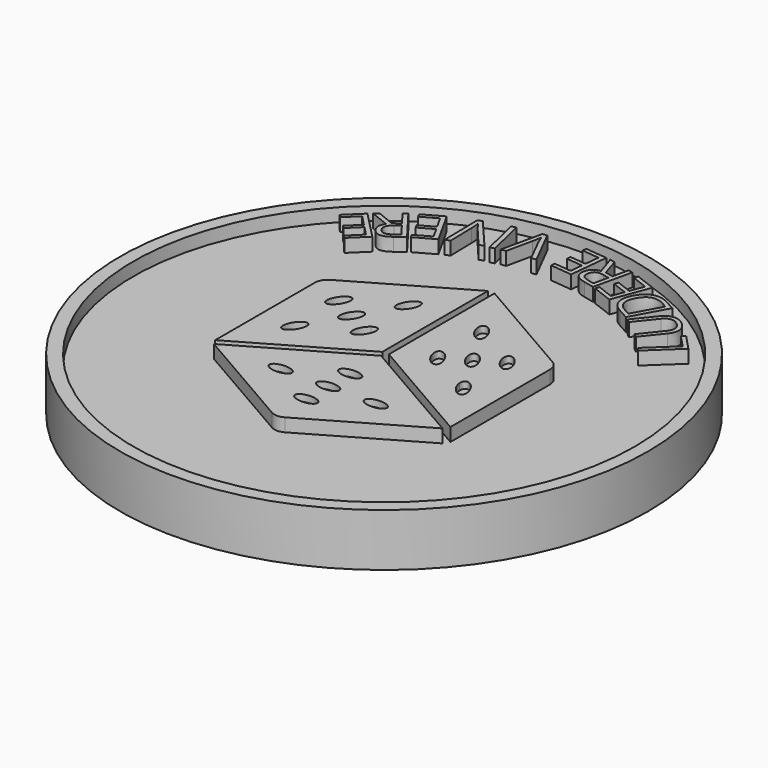
from build123d import *

# Parameters (mm, degrees)
F0_R          = 10
F1_DEPTH      = 2
F2_R          = 9.5
F3_DEPTH      = 0.5
F4_R          = 9.25
F5_DEPTH      = 0.5
F7_DEPTH      = 0.5
F9_DEPTH      = 0.25
F10_TEXT_SIZE = 2.0833333333
F11_DEPTH     = 0.5
F13_TEXT_SIZE = 15.2777777778
F14_DEPTH     = 0.5


# Not quite as in the source:
# - Text() gives the source's letters only with a copy of the font that has no kerning and outlines rounded to 1/6400 em; it was checked with that copy


with BuildPart() as f1:
    # F0 (on Top) → F1 (new body)
    with BuildSketch(Plane.XY):
        Circle(F0_R)
    extrude(amount=F1_DEPTH)

    # F2 (on face) → F3 (cut)
    with BuildSketch(Plane.XY.offset(2)):
        Circle(F2_R)
    extrude(amount=-F3_DEPTH, mode=Mode.SUBTRACT)

    # F4 (on face) → F5 (cut)
    with BuildSketch(Plane(origin=(0, 0, 0), x_dir=(1, 0, 0), z_dir=(0, 0, -1))):
        Circle(F4_R)
    extrude(amount=-F5_DEPTH, mode=Mode.SUBTRACT)

    # F6 (on face) → F7 (join, through all)
    with BuildSketch(Plane.XY.offset(2)):
        with BuildLine():
            Line((-0.125, 0.0721687836), (-0.125, 5.0721687836))
            Line((-0.125, 5.0721687836), (-4.2051270189, 2.7165063509))
            ThreePointArc((-4.2051270189, 2.7165063509), (-4.3881397208, 2.5334936491), (-4.4551270189, 2.2834936491))
            Line((-4.4551270189, 2.2834936491), (-4.4551270189, -2.4278312164))
            Line((-4.4551270189, -2.4278312164), (-0.125, 0.0721687836))
        make_face()
        with BuildLine():
            Line((0, -0.1443375673), (-4.3301270189, -2.6443375673))
            Line((-4.3301270189, -2.6443375673), (-0.25, -5))
            ThreePointArc((-0.25, -5), (0, -5.0669872981), (0.25, -5))
            Line((0.25, -5), (4.3301270189, -2.6443375673))
            Line((4.3301270189, -2.6443375673), (0, -0.1443375673))
        make_face()
        with BuildLine():
            Line((0.125, 0.0721687836), (4.4551270189, -2.4278312164))
            Line((4.4551270189, -2.4278312164), (4.4551270189, 2.2834936491))
            ThreePointArc((4.4551270189, 2.2834936491), (4.3881397208, 2.5334936491), (4.2051270189, 2.7165063509))
            Line((4.2051270189, 2.7165063509), (0.125, 5.0721687836))
            Line((0.125, 5.0721687836), (0.125, 0.0721687836))
        make_face()
    extrude(amount=-F7_DEPTH)

    # F8 (on face) → F9 (cut)
    with BuildSketch(Plane.XY.offset(2)):
        with BuildLine():
            add(Edge.make_bspline(
                [(-0.4265724856, -2.6443375673), (-0.4265724856, -3.0189013437), (0.2132862428, -2.8316194555), (0.8531449712, -2.6443375673), (0.2132862428, -2.4570556791), (-0.4265724856, -2.2697737909), (-0.4265724856, -2.6443375673)],
                knots=[0, 0, 0, 2.0943951024, 2.0943951024, 4.1887902048, 4.1887902048, 6.2831853072, 6.2831853072, 6.2831853072], degree=2, weights=[1, 0.5, 1, 0.5, 1, 0.5, 1]))
        make_face()
        with BuildLine():
            add(Edge.make_bspline(
                [(1.3734275144, -2.6443375673), (1.3734275144, -3.0189013437), (2.0132862428, -2.8316194555), (2.6531449712, -2.6443375673), (2.0132862428, -2.4570556791), (1.3734275144, -2.2697737909), (1.3734275144, -2.6443375673)],
                knots=[0, 0, 0, 2.0943951024, 2.0943951024, 4.1887902048, 4.1887902048, 6.2831853072, 6.2831853072, 6.2831853072], degree=2, weights=[1, 0.5, 1, 0.5, 1, 0.5, 1]))
        make_face()
        with BuildLine():
            add(Edge.make_bspline(
                [(-1.5185417438, -2.4818375673), (-2.2265724856, -2.1666585057), (-2.2265724856, -2.6443375673)],
                knots=[3.9918185291, 3.9918185291, 3.9918185291, 6.2831853072, 6.2831853072, 6.2831853072], degree=2, weights=[1, 0.4124236698, 1]))
            add(Edge.make_bspline(
                [(-2.2265724856, -2.6443375673), (-2.2265724856, -2.9796236254), (-1.6240714101, -2.8413437189), (-1.0215703345, -2.7030638124), (-1.5185417438, -2.4818375673)],
                knots=[0, 0, 0, 1.9959092646, 1.9959092646, 3.9918185291, 3.9918185291, 3.9918185291], degree=2, weights=[1, 0.5420222921, 1, 0.5420222921, 1]))
        make_face()
        with BuildLine():
            add(Edge.make_bspline(
                [(-0.4265724856, -1.6051070828), (-0.4265724856, -1.7030096523), (-0.2814582562, -1.7676070828)],
                knots=[0, 0, 0, 0.8502258755, 0.8502258755, 0.8502258755], degree=2, weights=[1, 0.9109921606, 1]))
            add(Edge.make_bspline(
                [(-0.2814582562, -1.7676070828), (0.1270605196, -1.9494587409), (0.378292689, -1.705041847), (0.6295248585, -1.460624953), (0.1014761864, -1.3950606558), (-0.4265724856, -1.3294963586), (-0.4265724856, -1.6051070828)],
                knots=[0.8502258755, 0.8502258755, 0.8502258755, 2.6612123527, 2.6612123527, 4.47219883, 4.47219883, 6.2831853072, 6.2831853072, 6.2831853072], degree=2, weights=[1, 0.6172976096, 1, 0.6172976096, 1, 0.6172976096, 1]))
        make_face()
        with BuildLine():
            add(Edge.make_bspline(
                [(-0.4265724856, -3.6835680518), (-0.4265724856, -4.0581318282), (0.2132862428, -3.87084994), (0.8531449712, -3.6835680518), (0.2132862428, -3.4962861636), (-0.4265724856, -3.3090042754), (-0.4265724856, -3.6835680518)],
                knots=[0, 0, 0, 2.0943951024, 2.0943951024, 4.1887902048, 4.1887902048, 6.2831853072, 6.2831853072, 6.2831853072], degree=2, weights=[1, 0.5, 1, 0.5, 1, 0.5, 1]))
        make_face()
        with BuildLine():
            add(Edge.make_bspline(
                [(1.6033497523, 0.4331309323), (1.6881358645, 0.482082217), (1.6715217657, 0.6400535414)],
                knots=[0, 0, 0, 0.8502258755, 0.8502258755, 0.8502258755], degree=2, weights=[1, 0.9109921606, 1]))
            add(Edge.make_bspline(
                [(1.6715217657, 0.6400535414), (1.6247505334, 1.0847670082), (1.2874632095, 1.1801320022), (0.9501758855, 1.2754969962), (1.1574198745, 0.7854112832), (1.3646638636, 0.2953255702), (1.6033497523, 0.4331309323)],
                knots=[0.8502258755, 0.8502258755, 0.8502258755, 2.6612123527, 2.6612123527, 4.47219883, 4.47219883, 6.2831853072, 6.2831853072, 6.2831853072], degree=2, weights=[1, 0.6172976096, 1, 0.6172976096, 1, 0.6172976096, 1]))
        make_face()
        with BuildLine():
            add(Edge.make_bspline(
                [(3.4033497523, -0.6060995522), (3.6937159961, -0.4384565232), (3.2727115465, 0.0141847608), (2.8517070968, 0.4668260447), (2.9086052532, -0.0741769432)],
                knots=[0, 0, 0, 1.9959092646, 1.9959092646, 3.9918185291, 3.9918185291, 3.9918185291], degree=2, weights=[1, 0.5420222921, 1, 0.5420222921, 1]))
            add(Edge.make_bspline(
                [(2.9086052532, -0.0741769432), (2.98966755, -0.844939083), (3.4033497523, -0.6060995522)],
                knots=[3.9918185291, 3.9918185291, 3.9918185291, 6.2831853072, 6.2831853072, 6.2831853072], degree=2, weights=[1, 0.4124236698, 1]))
        make_face()
        with BuildLine():
            add(Edge.make_bspline(
                [(1.6033497523, 2.5115919014), (1.9277314979, 2.6988737896), (1.4456112609, 3.1593667591), (0.9634910239, 3.6198597286), (1.1212295152, 2.9720848709), (1.2789680066, 2.3243100132), (1.6033497523, 2.5115919014)],
                knots=[0, 0, 0, 2.0943951024, 2.0943951024, 4.1887902048, 4.1887902048, 6.2831853072, 6.2831853072, 6.2831853072], degree=2, weights=[1, 0.5, 1, 0.5, 1, 0.5, 1]))
        make_face()
        with BuildLine():
            add(Edge.make_bspline(
                [(3.4033497523, 1.4723614168), (3.7277314979, 1.659643305), (3.2456112609, 2.1201362746), (2.7634910239, 2.5806292441), (2.9212295152, 1.9328543864), (3.0789680066, 1.2850795286), (3.4033497523, 1.4723614168)],
                knots=[0, 0, 0, 2.0943951024, 2.0943951024, 4.1887902048, 4.1887902048, 6.2831853072, 6.2831853072, 6.2831853072], degree=2, weights=[1, 0.5, 1, 0.5, 1, 0.5, 1]))
        make_face()
        with BuildLine():
            add(Edge.make_bspline(
                [(2.5033497523, 0.9527461746), (2.8277314979, 1.1400280628), (2.3456112609, 1.6005210323), (1.8634910239, 2.0610140018), (2.0212295152, 1.4132391441), (2.1789680066, 0.7654642864), (2.5033497523, 0.9527461746)],
                knots=[0, 0, 0, 2.0943951024, 2.0943951024, 4.1887902048, 4.1887902048, 6.2831853072, 6.2831853072, 6.2831853072], degree=2, weights=[1, 0.5, 1, 0.5, 1, 0.5, 1]))
        make_face()
        with BuildLine():
            add(Edge.make_bspline(
                [(-1.1767772667, 1.1719761505), (-1.2615633789, 1.2209274352), (-1.3900635095, 1.1275535414)],
                knots=[0, 0, 0, 0.8502258755, 0.8502258755, 0.8502258755], degree=2, weights=[1, 0.9109921606, 1]))
            add(Edge.make_bspline(
                [(-1.3900635095, 1.1275535414), (-1.751811053, 0.8646917327), (-1.6657558985, 0.5249098447), (-1.5797007439, 0.1851279568), (-1.258896061, 0.6096493726), (-0.938091378, 1.0341707884), (-1.1767772667, 1.1719761505)],
                knots=[0.8502258755, 0.8502258755, 0.8502258755, 2.6612123527, 2.6612123527, 4.47219883, 4.47219883, 6.2831853072, 6.2831853072, 6.2831853072], degree=2, weights=[1, 0.6172976096, 1, 0.6172976096, 1, 0.6172976096, 1]))
        make_face()
        with BuildLine():
            add(Edge.make_bspline(
                [(-1.1767772667, 3.2504371195), (-1.4671435105, 3.4180801486), (-1.6486401364, 2.8271589581), (-1.8301367623, 2.2362377676), (-1.3900635095, 2.5560145105)],
                knots=[0, 0, 0, 1.9959092646, 1.9959092646, 3.9918185291, 3.9918185291, 3.9918185291], degree=2, weights=[1, 0.5420222921, 1, 0.5420222921, 1]))
            add(Edge.make_bspline(
                [(-1.3900635095, 2.5560145105), (-0.7630950645, 3.0115975887), (-1.1767772667, 3.2504371195)],
                knots=[3.9918185291, 3.9918185291, 3.9918185291, 6.2831853072, 6.2831853072, 6.2831853072], degree=2, weights=[1, 0.4124236698, 1]))
        make_face()
        with BuildLine():
            add(Edge.make_bspline(
                [(-2.9767772667, 0.1327456659), (-3.3011590124, 0.3200275541), (-3.4588975037, -0.3277473036), (-3.6166359951, -0.9755221613), (-3.134515758, -0.5150291918), (-2.652395521, -0.0545362223), (-2.9767772667, 0.1327456659)],
                knots=[0, 0, 0, 2.0943951024, 2.0943951024, 4.1887902048, 4.1887902048, 6.2831853072, 6.2831853072, 6.2831853072], degree=2, weights=[1, 0.5, 1, 0.5, 1, 0.5, 1]))
        make_face()
        with BuildLine():
            add(Edge.make_bspline(
                [(-2.9767772667, 2.211206635), (-3.3011590124, 2.3984885232), (-3.4588975037, 1.7507136655), (-3.6166359951, 1.1029388078), (-3.134515758, 1.5634317773), (-2.652395521, 2.0239247468), (-2.9767772667, 2.211206635)],
                knots=[0, 0, 0, 2.0943951024, 2.0943951024, 4.1887902048, 4.1887902048, 6.2831853072, 6.2831853072, 6.2831853072], degree=2, weights=[1, 0.5, 1, 0.5, 1, 0.5, 1]))
        make_face()
        with BuildLine():
            add(Edge.make_bspline(
                [(-2.0767772667, 1.6915913927), (-2.4011590124, 1.8788732809), (-2.5588975037, 1.2310984232), (-2.7166359951, 0.5833235655), (-2.234515758, 1.043816535), (-1.752395521, 1.5043095045), (-2.0767772667, 1.6915913927)],
                knots=[0, 0, 0, 2.0943951024, 2.0943951024, 4.1887902048, 4.1887902048, 6.2831853072, 6.2831853072, 6.2831853072], degree=2, weights=[1, 0.5, 1, 0.5, 1, 0.5, 1]))
        make_face()
    extrude(amount=-F9_DEPTH, mode=Mode.SUBTRACT)

    # F10 (on face) → F11 (join, through all)
    with BuildSketch(Plane.XY.offset(2)):
        with Locations(Location((1.4901733322, 8.8949874364), (0, 0, 174.204199698))):
            Text('E', F10_TEXT_SIZE, font='Open Sans', text_align=(TextAlign.LEFT, TextAlign.BOTTOM))
        with Locations(Location((6.9602849105, 5.7354905649), (0, 0, 133.204199698))):
            Text('L', F10_TEXT_SIZE, font='Open Sans', text_align=(TextAlign.LEFT, TextAlign.BOTTOM))
        with Locations(Location((6.2088700096, 6.5562723689), (0, 0, 141.204199698))):
            Text('U', F10_TEXT_SIZE, font='Open Sans', text_align=(TextAlign.LEFT, TextAlign.BOTTOM))
        with Locations(Location((5.0041574298, 7.5193820274), (0, 0, 151.204199698))):
            Text('D', F10_TEXT_SIZE, font='Open Sans', text_align=(TextAlign.LEFT, TextAlign.BOTTOM))
        with Locations(Location((3.7415890618, 8.2062128505), (0, 0, 159.204199698))):
            Text('E', F10_TEXT_SIZE, font='Open Sans', text_align=(TextAlign.LEFT, TextAlign.BOTTOM))
        with Locations(Location((2.6697508212, 8.6228550543), (0, 0, 167.204199698))):
            Text('R', F10_TEXT_SIZE, font='Open Sans', text_align=(TextAlign.LEFT, TextAlign.BOTTOM))
        with Locations(Location((-0.4465810448, 9.0151662004), (0, 0, -172.795800302))):
            Text('V', F10_TEXT_SIZE, font='Open Sans', text_align=(TextAlign.LEFT, TextAlign.BOTTOM))
        with Locations(Location((-1.8063881617, 8.8205777878), (0, 0, -166.795800302))):
            Text('I', F10_TEXT_SIZE, font='Open Sans', text_align=(TextAlign.LEFT, TextAlign.BOTTOM))
        with Locations(Location((-2.5387907289, 8.6618241661), (0, 0, -159.295800302))):
            Text('V', F10_TEXT_SIZE, font='Open Sans', text_align=(TextAlign.LEFT, TextAlign.BOTTOM))
        with Locations(Location((-3.8812766637, 8.1410754519), (0, 0, -150.795800302))):
            Text('E', F10_TEXT_SIZE, font='Open Sans', text_align=(TextAlign.LEFT, TextAlign.BOTTOM))
        with Locations(Location((-4.8894074494, 7.5878121701), (0, 0, -142.795800302))):
            Text('R', F10_TEXT_SIZE, font='Open Sans', text_align=(TextAlign.LEFT, TextAlign.BOTTOM))
        with Locations(Location((-5.856090743, 6.8591267129), (0, 0, -135.795800302))):
            Text('E', F10_TEXT_SIZE, font='Open Sans', text_align=(TextAlign.LEFT, TextAlign.BOTTOM))
    extrude(amount=-F11_DEPTH)

    # F13 (on offset) → F14 (join, through all)
    with BuildSketch(Plane(origin=(0, 0, 0), x_dir=(1, 0, 0), z_dir=(0, 0, -1))):
        with Locations((-4.4233940972, -5.5)):
            Text('5', F13_TEXT_SIZE, font='Open Sans', text_align=(TextAlign.LEFT, TextAlign.BOTTOM))
    extrude(amount=-F14_DEPTH)


solid = f1.part
